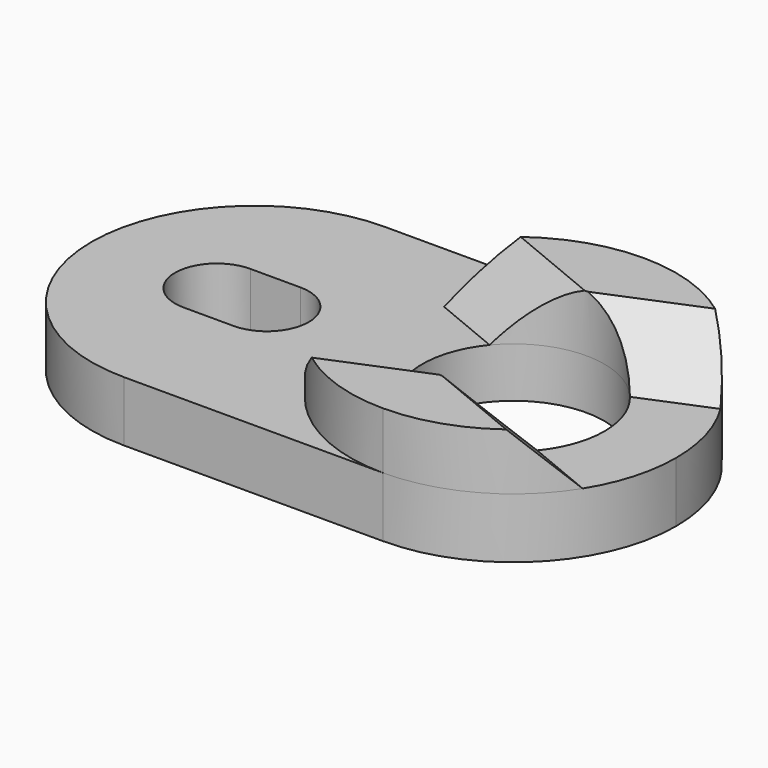
from build123d import *

# Parameters (mm, degrees)
F0_R        = 5.45
F1_DEPTH    = 3.6
F3_DEPTH    = 3.4
F4_T4_DEPTH = 30.0168298797
F5_T4_DEPTH = 28.3957620677
F6_T4_DEPTH = 30.0168298797
F7_T4_DEPTH = 28.3957620678
F8_R        = 7.5
F9_DEPTH    = 0.6


# Not quite as in the source:
# - a fillet or chamfer that OpenCascade refuses, or shapes differently, is made with other operations: its cross-section is extruded or revolved along the edge and cut away or added


with BuildPart() as f1:
    # F0 (on Top) → F1 (new body)
    with BuildSketch(Plane.XY):
        with BuildLine():
            Line((15.25, 9.75), (-0.25, 9.75))
            ThreePointArc((-0.25, 9.75), (-7.1442911166, 6.8942911166), (-10, 0))
            ThreePointArc((-10, 0), (-7.1442911166, -6.8942911166), (-0.25, -9.75))
            Line((-0.25, -9.75), (15.25, -9.75))
            ThreePointArc((15.25, -9.75), (22.1442911166, -6.8942911166), (25, 0))
            ThreePointArc((25, 0), (22.1442911166, 6.8942911166), (15.25, 9.75))
        make_face()
        with BuildLine():
            ThreePointArc((-2.5, -2.5), (-5, 0), (-2.5, 2.5))
            Line((-2.5, 2.5), (0.5, 2.5))
            ThreePointArc((0.5, 2.5), (3, 0), (0.5, -2.5))
            Line((0.5, -2.5), (-2.5, -2.5))
        make_face(mode=Mode.SUBTRACT)
        with Locations((15.25, 0)):
            Circle(F0_R, mode=Mode.SUBTRACT)
    extrude(amount=F1_DEPTH)

    # F2 (on face) → F3 (join)
    with BuildSketch(Plane.XY.offset(3.6)):
        with BuildLine():
            Line((6.242174558, 3.7311634656), (10.2148565478, 2.0856247064))
            ThreePointArc((10.2148565478, 2.0856247064), (15.25, 5.45), (20.2851434522, 2.0856247064))
            Line((20.2851434522, 2.0856247064), (24.257825442, 3.7311634656))
            ThreePointArc((24.257825442, 3.7311634656), (20.6668097719, 8.1068287199), (15.25, 9.75))
            ThreePointArc((15.25, 9.75), (9.8331902281, 8.1068287199), (6.242174558, 3.7311634656))
        make_face()
        with BuildLine():
            ThreePointArc((20.2851434522, -2.0856247064), (15.25, -5.45), (10.2148565478, -2.0856247064))
            Line((10.2148565478, -2.0856247064), (6.242174558, -3.7311634656))
            ThreePointArc((6.242174558, -3.7311634656), (9.8331902281, -8.1068287199), (15.25, -9.75))
            ThreePointArc((15.25, -9.75), (20.6668097719, -8.1068287199), (24.257825442, -3.7311634656))
            Line((24.257825442, -3.7311634656), (20.2851434522, -2.0856247064))
        make_face()
    extrude(amount=F3_DEPTH)

    # F4: chamfer of 5 on 1 edges, made by hand


with BuildPart() as f4_tool2:
    # F4_s3 → F4_t4 (new body)
    with BuildSketch(Plane(origin=(-7.8707626189, 3.260176623, 0), x_dir=(0, 0, 1), z_dir=(0.9238795325, -0.3826834324, 0))):
        Polygon((2, -5.8359223436), (7, -10.8359223436), (7, -5.8359223436), align=None)
    extrude(amount=F4_T4_DEPTH)

    split(bisect_by=Plane.XY.offset(3.6), keep=Keep.TOP)


with BuildPart() as f1_1:
    add(f1.part)

    # F4_t1: cut F4_tool2
    add(f4_tool2.part, mode=Mode.SUBTRACT)

    # F5: chamfer of 5 on 1 edges, made by hand


with BuildPart() as f5_tool2:
    # F5_s3 → F5_t4 (new body)
    with BuildSketch(Plane(origin=(7.6698776475, 3.1769673433, 0), x_dir=(0, 0, 1), z_dir=(0.9238795325, 0.3826834324, 0))):
        Polygon((2, 5.8359223436), (7, 0.8359223436), (7, 5.8359223436), align=None)
    extrude(amount=F5_T4_DEPTH)

    split(bisect_by=Plane.XY.offset(3.6), keep=Keep.TOP)


with BuildPart() as f1_2:
    add(f1_1.part)

    # F5_t1: cut F5_tool2
    add(f5_tool2.part, mode=Mode.SUBTRACT)

    # F6: chamfer of 5 on 1 edges, made by hand


with BuildPart() as f6_tool2:
    # F6_s3 → F6_t4 (new body)
    with BuildSketch(Plane(origin=(6.1722062753, -2.556611549, 0), x_dir=(0, 0, 1), z_dir=(0.9238795325, -0.3826834324, 0))):
        Polygon((2, -5.8359223436), (7, -0.8359223436), (7, -5.8359223436), align=None)
    extrude(amount=F6_T4_DEPTH)

    split(bisect_by=Plane.XY.offset(3.6), keep=Keep.TOP)


with BuildPart() as f1_3:
    add(f1_2.part)

    # F6_t1: cut F6_tool2
    add(f6_tool2.part, mode=Mode.SUBTRACT)

    # F7: chamfer of 5 on 1 edges, made by hand


with BuildPart() as f7_tool2:
    # F7_s3 → F7_t4 (new body)
    with BuildSketch(Plane(origin=(18.3635007657, 7.6064110698, 0), x_dir=(0, 0, 1), z_dir=(-0.9238795325, -0.3826834324, 0))):
        Polygon((7, -10.8359223436), (2, -5.8359223436), (7, -5.8359223436), align=None)
    extrude(amount=F7_T4_DEPTH)

    split(bisect_by=Plane.XY.offset(3.6), keep=Keep.TOP)


with BuildPart() as f1_4:
    add(f1_3.part)

    # F7_t1: cut F7_tool2
    add(f7_tool2.part, mode=Mode.SUBTRACT)

    # F8 (on face) → F9 (cut)
    with BuildSketch(Plane(origin=(0, 0, 0), x_dir=(1, 0, 0), z_dir=(0, 0, -1))):
        with Locations((15.25, 0)):
            Circle(F8_R)
    extrude(amount=-F9_DEPTH, mode=Mode.SUBTRACT)


solid = f1_4.part
